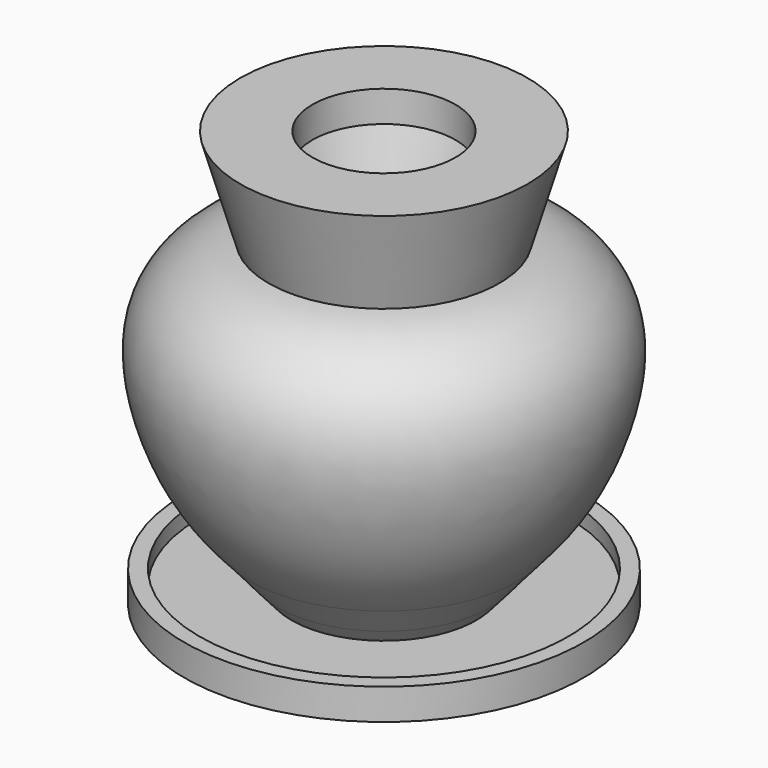
from build123d import *


# Not quite as in the source:
# - ends of sketch curves that miss each other by under 0.0002 mm in the source are joined
# - the dataset's text gives a spline's control points without its knots; the knots are read off the source's solid


with BuildPart() as f2:
    # F0 (on Front) → F2 (revolve)
    with BuildSketch(Plane.XZ):
        with BuildLine():
            Line((-25.0346597179, 47.2444333136), (-17.5361242145, 47.2444333136))
            Line((-17.5361242145, 47.2444333136), (-17.5361242145, 54.8644333136))
            Line((-17.5361242145, 54.8644333136), (-35.2048012345, 54.8644333136))
            Line((-35.2048012345, 54.8644333136), (-28.289489922, 31.2389873851))
            add(Edge.make_bspline(
                [(-28.289489922, 31.2389873851), (-28.6041178305, 31.2124391794), (-29.5101526308, 31.1204722173), (-31.0376869866, 30.8857881394), (-32.5710309425, 30.5302540963), (-33.8104853839, 30.1596233424), (-35.03305031, 29.7369084446), (-36.5259601871, 29.1148051851), (-38.2561233277, 28.2232253901), (-40.4719095091, 26.8452842687), (-43.0513465812, 24.7723455812), (-45.3030601154, 22.2301415304), (-46.8411309798, 19.9149750587), (-47.6750154356, 18.3527943026), (-48.2539627145, 17.0386598282), (-48.7710780187, 15.6785979349), (-49.2747924885, 13.9684627304), (-49.6809009584, 11.9193903816), (-49.9924653672, 9.2097291865), (-50.014170035, 5.8826420041), (-49.6087574786, 2.0063972781), (-48.8840460528, -1.7439824698), (-48.1669934508, -4.4469548009), (-47.6395734534, -6.1946719725), (-47.2769511646, -7.3423598376), (-46.6080410139, -9.3297961071), (-45.5428226338, -12.1255090134), (-44.0727014161, -15.4095578979), (-42.3954025631, -18.6253966268), (-40.8154347549, -21.2492307316), (-39.4379157767, -23.3161012552), (-38.3467370235, -24.8512380934), (-37.1981355099, -26.3706166271), (-35.9856097961, -27.8814076992), (-34.733175354, -29.3578025206), (-33.6086751998, -30.6252778512), (-32.9054955981, -31.393909129), (-32.6284556557, -31.6935088743)],
                knots=[0.1165840616, 0.1165840616, 0.1165840616, 0.1165840616, 0.125, 0.140625, 0.15625, 0.1640625, 0.171875, 0.1875, 0.203125, 0.21875, 0.25, 0.28125, 0.296875, 0.3125, 0.3203125, 0.328125, 0.34375, 0.359375, 0.375, 0.40625, 0.4375, 0.46875, 0.5, 0.5078125, 0.515625, 0.53125, 0.5625, 0.59375, 0.625, 0.65625, 0.671875, 0.6875, 0.703125, 0.71875, 0.734375, 0.75, 0.7601763788, 0.7601763788, 0.7601763788, 0.7601763788], degree=3))
            add(Edge.make_bspline(
                [(-32.6284556557, -31.6935088743), (-29.3537211027, -35.1977835064), (-28.2000626357, -37.0205005319), (-25.8868339521, -39.5605005324)],
                knots=[0, 0, 0, 0, 10.3604556265, 10.3604556265, 10.3604556265, 10.3604556265], degree=3))
            Line((-25.8868339521, -39.5605005324), (-14.9648338556, -39.5605005324))
            add(Edge.make_bspline(
                [(-17.928166315, 22.9658335447), (-22.4574145842, 23.6269687071), (-31.577565005, 24.9328482979), (-44.3360106306, 14.4436354704), (-40.900346724, -5.6664430766), (-32.2079032901, -22.4117926186), (-17.1962934677, -36.0765255771), (-16.5069680661, -37.3918637633), (-14.9648338556, -39.5605005324)],
                knots=[0, 0, 0, 0, 0.1614458367, 0.3246949128, 0.5143949366, 0.71498079, 0.9025327716, 1, 1, 1, 1], degree=3))
            Line((-17.928166315, 22.9658335447), (-25.0346597179, 47.2444333136))
        make_face()
        Polygon((0, -39.5605005324), (-14.9648338556, -39.5605005324), (-8.756195195, -47.1805005324), (0, -47.1805005324), (0, -44.1324982991), align=None)
        Polygon((-8.756195195, -47.1805005324), (-14.9648338556, -39.5605005324), (-25.8868339521, -39.5605005324), (-19.2331615835, -47.1805005324), align=None)
    revolve(axis=Axis((0, 0, 8.1670787185), (0, 0, 1)))

    # F1 (on Front) → F3 (revolve)
    with BuildSketch(Plane.XZ):
        Polygon((-48.2781451661, -39.4817550206), (-48.9660029811, -39.4817550206), (-48.9660029811, -47.1017550206), (0, -47.1017550206), (0, -43.2917550206), (-45.1560029811, -43.2917550206), (-45.1560029811, -39.4817550206), align=None)
    revolve(axis=Axis((0, 0, -41.8464994157), (0, 0, -1)))


solid = f2.part
